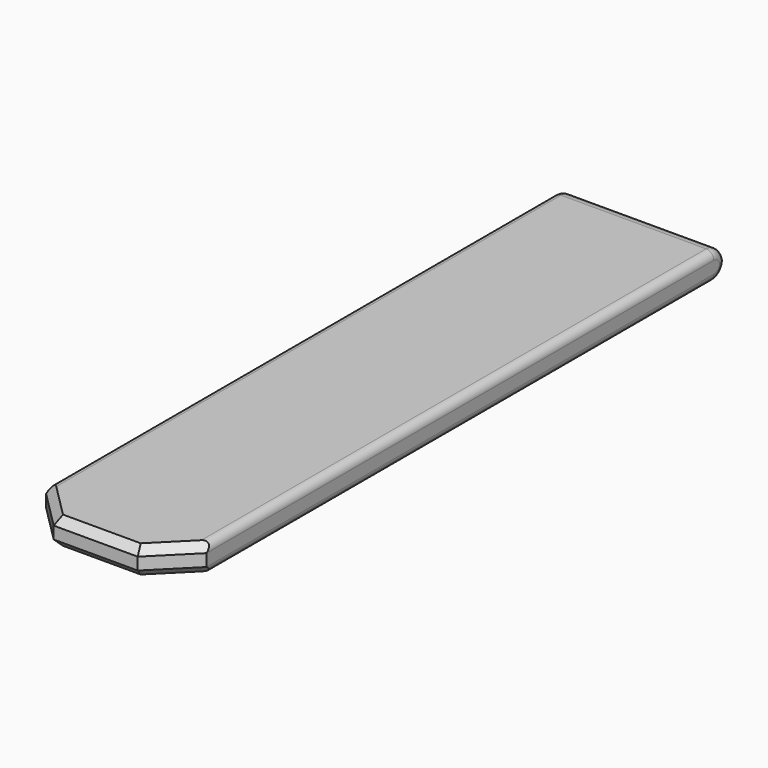
from build123d import *

# Parameters (mm, degrees)
F0_W         = 10.5
F0_H         = 45
F1_DEPTH     = 1.8
F2_SIZE      = 2.5
F3_SIZE      = 0.5
F4_T1_DEPTH  = 15.5
F5_T1_DEPTH  = 42.0428932188
F5_T4_ANGLE  = 155.9057709944
F5_T6_ANGLE  = 155.9057709944
F5_T8_ANGLE  = 155.9057709944
F5_T10_ANGLE = 155.9057709944


# Not quite as in the source:
# - a fillet or chamfer that OpenCascade refuses, or shapes differently, is made with other operations: its cross-section is extruded or revolved along the edge and cut away or added


with BuildPart() as f1:
    # F0 (on Top) → F1 (new body)
    with BuildSketch(Plane.XY):
        Rectangle(F0_W, F0_H)
    extrude(amount=F1_DEPTH)

    # F2
    f2_edges = [f1.edges().sort_by_distance(p)[0] for p in [
        (5.25, -22.5, 0.9),
        (-5.25, -22.5, 0.9),
    ]]
    chamfer(f2_edges, length=F2_SIZE)

    # F3
    f3_edges = [f1.edges().sort_by_distance(p)[0] for p in [
        (0, -22.5, 1.8),
        (4, -21.25, 1.8),
        (4, -21.25, 0),
        (0, -22.5, 0),
        (-4, -21.25, 1.8),
        (-4, -21.25, 0),
    ]]
    chamfer(f3_edges, length=F3_SIZE)

    # F4: fillet of radius 1 on 2 edges, made by hand

    # F4_s2 → F4_t1 (cut)
    with BuildSketch(Plane.YZ.offset(-7.75)):
        with BuildLine():
            ThreePointArc((21.5, 0), (22.2071067812, 0.2928932188), (22.5, 1))
            Line((22.5, 1), (22.5, 0))
            Line((22.5, 0), (21.5, 0))
        make_face()
        with BuildLine():
            ThreePointArc((21.5, 1.8), (22.2071067812, 1.5071067812), (22.5, 0.8))
            Line((22.5, 0.8), (22.5, 1.8))
            Line((22.5, 1.8), (21.5, 1.8))
        make_face()
    extrude(amount=F4_T1_DEPTH, mode=Mode.SUBTRACT)

    # F5: fillet of radius 0.5 on 8 edges, made by hand

    # F5_s2 → F5_t1 (cut)
    with BuildSketch(Plane.XZ.offset(-21.5)):
        with BuildLine():
            ThreePointArc((4.75, 1.8), (5.1035533906, 1.6535533906), (5.25, 1.3))
            Line((5.25, 1.3), (5.25, 1.8))
            Line((5.25, 1.8), (4.75, 1.8))
        make_face()
        with BuildLine():
            ThreePointArc((4.75, 0), (5.1035533906, 0.1464466094), (5.25, 0.5))
            Line((5.25, 0.5), (5.25, 0))
            Line((5.25, 0), (4.75, 0))
        make_face()
        with BuildLine():
            ThreePointArc((-5.25, 1.3), (-5.1035533906, 1.6535533906), (-4.75, 1.8))
            Line((-4.75, 1.8), (-5.25, 1.8))
            Line((-5.25, 1.8), (-5.25, 1.3))
        make_face()
        with BuildLine():
            ThreePointArc((-5.25, 0.5), (-5.1035533906, 0.1464466094), (-4.75, 0))
            Line((-4.75, 0), (-5.25, 0))
            Line((-5.25, 0), (-5.25, 0.5))
        make_face()
    extrude(amount=F5_T1_DEPTH, mode=Mode.SUBTRACT)

    # F5_s3 → F5_t4 (revolve, cut)
    with BuildSketch(Plane.XZ.offset(-21.5)):
        with BuildLine():
            ThreePointArc((-5.25, 1.3), (-5.1035533906, 1.6535533906), (-4.75, 1.8))
            Line((-4.75, 1.8), (-5.25, 1.8))
            Line((-5.25, 1.8), (-5.25, 1.3))
        make_face()
    revolve(axis=Axis((-5.25, 21.5, 0.8), (-1, 0, 0)), revolution_arc=F5_T4_ANGLE, mode=Mode.SUBTRACT)

    # F5_s5 → F5_t6 (revolve, cut)
    with BuildSketch(Plane(origin=(0, 17.5441674109, -7.8457647459), x_dir=(1, 0, 0), z_dir=(0, -0.9128753008, 0.4082385151))):
        with BuildLine():
            ThreePointArc((-5.25, 10.1900033752), (-5.1035533906, 10.5435567657), (-4.75, 10.6900033752))
            Line((-4.75, 10.6900033752), (-5.25, 10.6900033752))
            Line((-5.25, 10.6900033752), (-5.25, 10.1900033752))
        make_face()
    revolve(axis=Axis((-5.25, 21.5, 1), (-1, 0, 0)), revolution_arc=F5_T6_ANGLE, mode=Mode.SUBTRACT)

    # F5_s7 → F5_t8 (revolve, cut)
    with BuildSketch(Plane(origin=(0, 17.5441674109, -7.8457647459), x_dir=(1, 0, 0), z_dir=(0, -0.9128753008, 0.4082385151))):
        with BuildLine():
            ThreePointArc((5.25, 10.1900033752), (5.1035533906, 10.5435567657), (4.75, 10.6900033752))
            Line((4.75, 10.6900033752), (5.25, 10.6900033752))
            Line((5.25, 10.6900033752), (5.25, 10.1900033752))
        make_face()
    revolve(axis=Axis((5.25, 21.5, 1), (-1, 0, 0)), revolution_arc=F5_T8_ANGLE, mode=Mode.SUBTRACT)

    # F5_s9 → F5_t10 (revolve, cut)
    with BuildSketch(Plane.XZ.offset(-21.5)):
        with BuildLine():
            ThreePointArc((5.25, 1.3), (5.1035533906, 1.6535533906), (4.75, 1.8))
            Line((4.75, 1.8), (5.25, 1.8))
            Line((5.25, 1.8), (5.25, 1.3))
        make_face()
    revolve(axis=Axis((5.25, 21.5, 0.8), (-1, 0, 0)), revolution_arc=F5_T10_ANGLE, mode=Mode.SUBTRACT)


solid = f1.part
